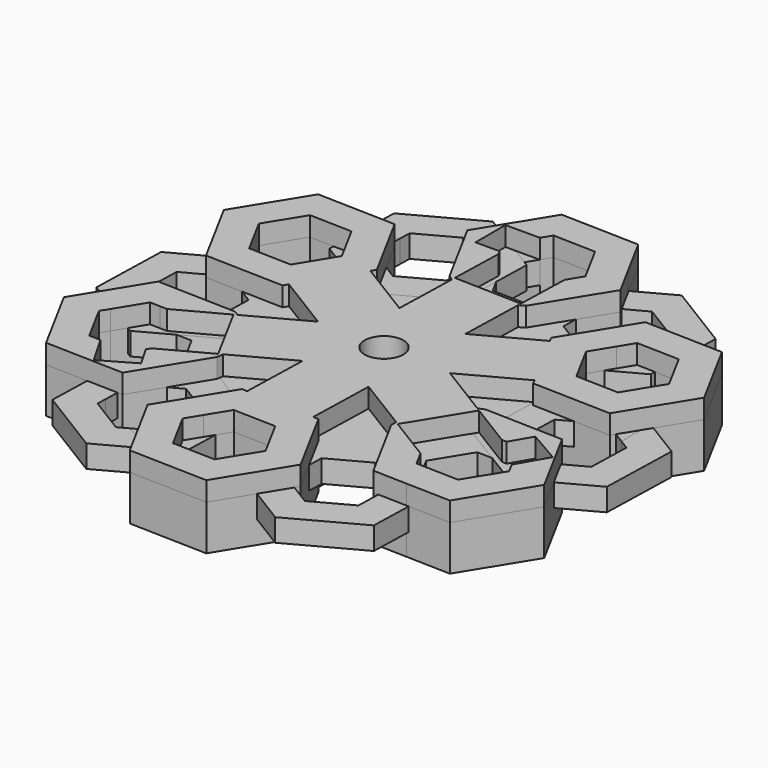
from build123d import *
from build123d import SkipClean  # not in build123d's __all__

# Parameters (mm, degrees)
F2_DEPTH      = 3.5
F0_R          = 3
F3_DEPTH      = 25.4
F3_DEPTH_BACK = 25.4
F4_COUNT      = 4
F5_DEPTH      = 7
F5_DEPTH_BACK = 3


with BuildPart() as f2:
    # F1 (on Top) → F2 (new body)
    with BuildSketch(Plane.XY):
        Polygon((-13.5901660179, 14.0965503932), (-8.9344304844, 5.4925473541), (0.2894702979, 10.4837174449), (-4.4172599299, 19.1819609111), (-7.8331099594, 13.2655351088), align=None)
        Polygon((0.2894702979, 10.4837174449), (-8.9344304844, 5.4925473541), (-9.2239007824, -4.9911700908), (-0.2894702979, -10.4837174449), (8.9344304844, -5.4925473541), (9.2239007824, 4.9911700908), align=None)
        Polygon((-9.2239007824, -4.9911700908), (-8.9344304844, 5.4925473541), (-19.33204223, 5.7796401517), (-19.6215125279, -4.7040772933), align=None)
        Polygon((5.7369058266, 19.3447669565), (0.2894702979, 10.4837174449), (9.2239007824, 4.9911700908), (14.671336311, 13.8522196024), align=None)
        Polygon((-0.2894702979, -10.4837174449), (-9.2239007824, -4.9911700908), (-14.4034354784, -13.4164397699), (-7.5717354193, -13.4164397699), (-5.4128877373, -18.8177042097), align=None)
        Polygon((-19.6215125279, -4.7040772933), (-19.33204223, 5.7796401517), (-27.5227283397, 6.0057966044), (-24.2015305745, 3.9640507953), (-24.3833960163, -2.6225521094), (-27.8121986377, -4.4779208405), align=None)
        Polygon((-27.5227283397, 6.0057966044), (-19.33204223, 5.7796401517), (-19.3090755972, 6.6114204417), (-29.661225172, 12.9755274607), (-40.3487783102, 7.1923564546), (-40.6841818737, -4.9549215704), (-30.3320322989, -11.3190285894), (-19.6444791607, -5.5358575833), (-19.6215125279, -4.7040772933), (-27.8121986377, -4.4779208405), (-30.1784941773, -5.758353469), (-35.7917268964, -2.307551924), (-35.6098614546, 4.2790509807), (-29.8147632936, 7.4148523403), align=None)
        Polygon((-14.6164328792, 14.2446892056), (-13.5901660179, 14.0965503932), (-13.8846067013, 14.6406896632), align=None)
        Polygon((-13.8846067013, 14.6406896632), (-13.5901660179, 14.0965503932), (-7.8331099594, 13.2655351088), (-4.4172599299, 19.1819609111), (-4.6607059189, 19.631859754), align=None)
        Polygon((19.0030537552, 4.7211538166), (9.2239007824, 4.9911700908), (8.9344304844, -5.4925473541), (18.8206954083, -5.7655211411), (15.4048453788, 0.1509046611), align=None)
        Polygon((10.0281061148, 26.3250309756), (5.7369058266, 19.3447669565), (14.671336311, 13.8522196024), (18.9625365992, 20.8324836215), (15.5337339778, 18.9771148903), (9.9205012587, 22.4279164353), align=None)
        Polygon((5.0280462814, 19.7805467889), (5.7369058266, 19.3447669565), (10.0281061148, 26.3250309756), (10.1023667005, 29.01451934), (15.8974648615, 32.1503206996), (21.5106975807, 28.6995191546), (21.3288321388, 22.1129162499), (18.9625365992, 20.8324836215), (14.671336311, 13.8522196024), (15.3801958562, 13.4164397699), (26.0677489945, 19.199610776), (26.4031525579, 31.346888801), (16.0510029831, 37.71099582), (5.3634498449, 31.9278248139), align=None)
        Polygon((-4.6607059189, 19.631859754), (-4.4172599299, 19.1819609111), (-3.928879741, 20.0278602116), align=None)
        Polygon((8.9344304844, -5.4925473541), (-0.2894702979, -10.4837174449), (4.6607059189, -19.631859754), (13.8846067013, -14.6406896632), align=None)
        Polygon((-7.5717354193, -13.4164397699), (-14.4034354784, -13.4164397699), (-14.671336311, -13.8522196024), (-5.7369058266, -19.3447669565), (-5.4128877373, -18.8177042097), align=None)
        Polygon((-14.671336311, -13.8522196024), (-14.4034354784, -13.4164397699), (-15.3801958562, -13.4164397699), align=None)
        Polygon((-14.6164328792, 14.2446892056), (-13.8846067013, 14.6406896632), (-17.7840925229, 21.8471101351), (-18.4276710544, 22.2427576883), (-21.6642116636, 20.3741400963), (-24.566763318, 25.4015070333), (-19.9431849809, 28.0709312309), (-19.8942620349, 29.8427687756), (-14.0991638739, 32.9785701353), (-12.8127146622, 32.1877101888), (-8.0689793759, 34.9265070333), (-13.9456257523, 38.5392452557), (-24.6331788906, 32.7560742496), (-24.968582454, 20.6087962246), align=None)
        Polygon((19.6444791607, 5.5358575833), (19.0030537552, 4.7211538166), (19.6215125279, 4.7040772933), align=None)
        Polygon((19.6215125279, 4.7040772933), (19.0030537552, 4.7211538166), (15.4048453788, 0.1509046611), (18.8206954083, -5.7655211411), (19.33204223, -5.7796401517), align=None)
        Polygon((-8.5601917405, 26.8382802259), (-4.6607059189, 19.631859754), (-3.928879741, 20.0278602116), (-3.5934761776, 32.1751382367), (-8.0689793759, 34.9265070333), (-5.1664277215, 29.8991400963), (-8.5292859282, 27.9575930054), align=None)
        Polygon((-5.0280462814, -19.7805467889), (-5.4128877373, -18.8177042097), (-5.7369058266, -19.3447669565), align=None)
        Polygon((8.5601917405, -26.8382802259), (4.6607059189, -19.631859754), (3.928879741, -20.0278602116), (3.5934761776, -32.1751382367), (13.9456257523, -38.5392452557), (24.6331788906, -32.7560742496), (24.968582454, -20.6087962246), (14.6164328792, -14.2446892056), (13.8846067013, -14.6406896632), (17.7840925229, -21.8471101351), (20.0761274768, -23.256165871), (19.8942620349, -29.8427687756), (14.0991638739, -32.9785701353), (8.4859311548, -29.5277685902), align=None)
        Polygon((13.8846067013, -14.6406896632), (4.6607059189, -19.631859754), (8.5601917405, -26.8382802259), (8.6677965966, -22.9411656856), (14.4628947576, -19.805364326), (17.7840925229, -21.8471101351), align=None)
        Polygon((-18.9625365992, -20.8324836215), (-14.671336311, -13.8522196024), (-15.3801958562, -13.4164397699), (-26.0677489945, -19.199610776), (-26.2127526683, -24.4511946388), (-23.3102010139, -19.4238277018), (-19.9473428072, -21.3653747927), align=None)
        Polygon((19.33204223, -5.7796401517), (18.8206954083, -5.7655211411), (19.3090755972, -6.6114204417), align=None)
        Polygon((19.6444791607, 5.5358575833), (19.6215125279, 4.7040772933), (27.8121986377, 4.4779208405), (28.4766287355, 4.8374524216), (28.4766287355, 8.5746876055), (34.2817320443, 8.5746876055), (34.2817320443, 3.2358392104), (35.7917268964, 2.307551924), (35.6098614546, -4.2790509807), (34.2817320443, -4.9977187055), (34.2817320443, -10.4753123945), (40.3487783102, -7.1923564546), (40.6841818737, 4.9549215704), (30.3320322989, 11.3190285894), align=None)
        Polygon((-5.0280462814, -19.7805467889), (-5.7369058266, -19.3447669565), (-10.0281061148, -26.3250309756), (-10.0489576811, -27.0802101098), (-6.8124170718, -28.9488277018), (-9.7149687263, -33.9761946388), (-14.3385470634, -31.3067704413), (-15.8974648615, -32.1503206996), (-21.5106975807, -28.6995191546), (-21.4690173821, -27.1899914833), (-26.2127526683, -24.4511946388), (-26.4031525579, -31.346888801), (-16.0510029831, -37.71099582), (-5.3634498449, -31.9278248139), align=None)
        Polygon((27.5227283397, -6.0057966044), (19.33204223, -5.7796401517), (19.3090755972, -6.6114204417), (29.661225172, -12.9755274607), (34.2817320443, -10.4753123945), (28.4766287355, -10.4753123945), (28.4766287355, -6.5922182127), align=None)
        Polygon((-8.4859311548, 29.5277685902), (-8.5292859282, 27.9575930054), (-5.1664277215, 29.8991400963), (-8.0689793759, 34.9265070333), (-12.8127146622, 32.1877101888), align=None)
        Polygon((-21.3288321388, -22.1129162499), (-19.9473428072, -21.3653747927), (-23.3102010139, -19.4238277018), (-26.2127526683, -24.4511946388), (-21.4690173821, -27.1899914833), align=None)
        Polygon((29.8147632936, -7.4148523403), (28.4766287355, -6.5922182127), (28.4766287355, -10.4753123945), (34.2817320443, -10.4753123945), (34.2817320443, -4.9977187055), align=None)
    extrude(amount=F2_DEPTH)

    # F0 (on Top) → F3 (cut, two sides)
    with BuildSketch(Plane.XY) as f3_sk:
        Circle(F0_R)
    extrude(amount=-F3_DEPTH, mode=Mode.SUBTRACT)
    extrude(f3_sk.sketch, amount=F3_DEPTH_BACK, mode=Mode.SUBTRACT)


with BuildPart() as f4_1:
    # F4: instance of F2
    add(f2.part.rotate(Axis((0, 0, 3.5), (0, 0, 1)), 1 * 360 / F4_COUNT), clean=False)


with BuildPart() as f4_2:
    # F4: instance of F2
    add(f2.part.rotate(Axis((0, 0, 3.5), (0, 0, 1)), 2 * 360 / F4_COUNT), clean=False)


with BuildPart() as f4_3:
    # F4: instance of F2
    add(f2.part.rotate(Axis((0, 0, 3.5), (0, 0, 1)), 3 * 360 / F4_COUNT), clean=False)


with BuildPart() as f2_1:
    add(f2.part, clean=False)

    # F5 (add, two sides): a face of the model
    f5_faces = [f4_1.part.faces().sort_by_distance(p)[0] for p in [
        (-14.2994437173, -3.0496329731, 3.5),
    ]]
    with SkipClean():  # cleaning this boolean's faces spoils the solid; the shape is the same uncleaned
        extrude(f5_faces, amount=-F5_DEPTH)
        extrude(f5_faces, amount=F5_DEPTH_BACK)


solid = Compound([f4_1.part, f4_2.part, f4_3.part, f2_1.part])
